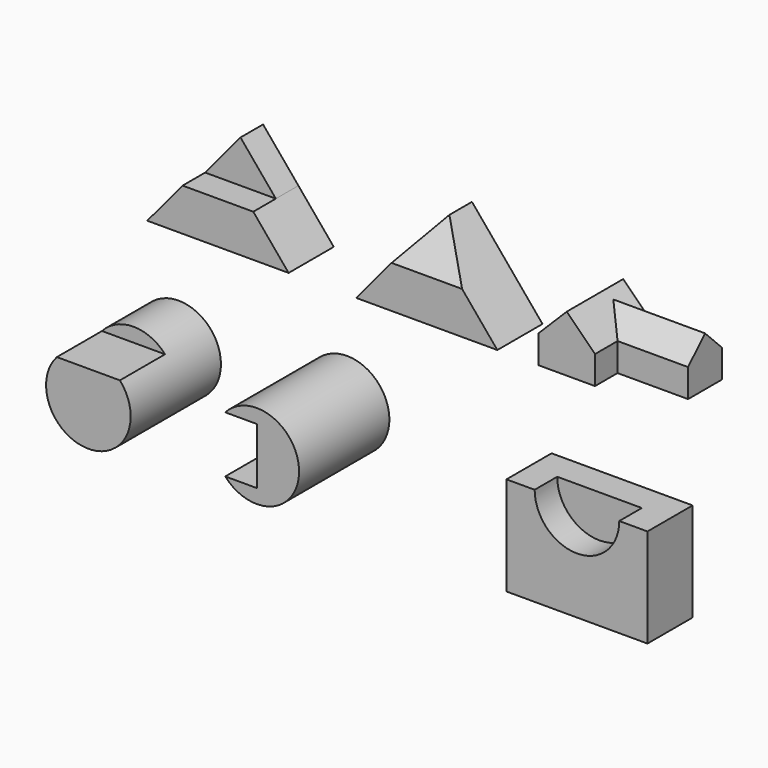
from build123d import *

# Parameters (mm, degrees)
F1_DEPTH  = 101.6
F2_DEPTH  = 50.8
F3_DEPTH  = 101.6
F7_DEPTH  = 63.5
F9_DEPTH  = 127
F12_DEPTH = 165.1
F13_R     = 76.2
F14_DEPTH = 203.2
F16_DEPTH = 101.6
F18_DEPTH = 203.2
F20_DEPTH = 101.6
F21_W     = 254
F21_H     = 177.8
F22_DEPTH = 101.6
F24_DEPTH = 50.8


with BuildPart() as f1:
    # F0 (on Front) → F1 (new body)
    with BuildSketch(Plane.XZ):
        Polygon((275.9973074218, 152.7659382395), (212.3448331553, 76.3829691198), (339.6497816883, 76.3829691198), align=None)
        Polygon((212.3448331553, 76.3829691198), (148.6923588888, 0), (403.3022559547, 0), (339.6497816883, 76.3829691198), align=None)
    extrude(amount=-F1_DEPTH)

    # F0 (on Front) → F2 (cut)
    with BuildSketch(Plane.XZ):
        Polygon((275.9973074218, 152.7659382395), (212.3448331553, 76.3829691198), (339.6497816883, 76.3829691198), align=None)
    extrude(amount=-F2_DEPTH, mode=Mode.SUBTRACT)


with BuildPart() as f3:
    # F0 (on Front) → F3 (new body)
    with BuildSketch(Plane.XZ):
        Polygon((652.2500761549, 152.4), (588.7500761549, 76.2), (715.7500761549, 76.2), align=None)
        Polygon((588.7500761549, 76.2), (525.2500761549, 0), (779.2500761549, 0), (715.7500761549, 76.2), align=None)
    extrude(amount=-F3_DEPTH)

    # F6 (on 3pt) → F7 (cut, symmetric)
    with BuildSketch(Plane.YZ.offset(652.2500761549)):
        Polygon((0, 152.4), (0, 76.2), (50.8, 152.4), align=None)
    extrude(amount=F7_DEPTH, both=True, mode=Mode.SUBTRACT)


with BuildPart() as f9:
    # F8 (on Front) → F9 (new body)
    with BuildSketch(Plane.XZ):
        Polygon((853.4919664163, 50.8), (853.4919664163, 0), (955.0919664163, 0), (955.0919664163, 50.8), (904.2919664163, 101.6), align=None)
    extrude(amount=-F9_DEPTH)

    # F11 (on offset) → F12 (join)
    with BuildSketch(Plane.YZ.offset(1082.0919664163)):
        Polygon((50.8, 0), (127, 0), (127, 50.8), (88.9, 88.9), (50.8, 50.8), align=None)
    extrude(amount=-F12_DEPTH)


with BuildPart() as f14:
    # F13 (on Front) → F14 (new body)
    with BuildSketch(Plane.XZ):
        with Locations((205.21299541, -184.5077127218)):
            Circle(F13_R)
    extrude(amount=F14_DEPTH)

    # F15 (on face) → F16 (cut)
    with BuildSketch(Plane.XZ.offset(203.2)):
        with BuildLine():
            Line((148.4525080283, -133.667894939), (202.7499394524, -133.667894939))
            Line((202.7499394524, -133.667894939), (261.9734827917, -133.667894939))
            ThreePointArc((261.9734827917, -133.667894939), (205.21299541, -108.3077127218), (148.4525080283, -133.667894939))
        make_face()
    extrude(amount=-F16_DEPTH, mode=Mode.SUBTRACT)


with BuildPart() as f18:
    # F17 (on Front) → F18 (new body)
    with BuildSketch(Plane.XZ):
        with BuildLine():
            ThreePointArc((451.7231056446, -224.286083746), (535.7090755138, -244.6700174989), (584.7192322731, -173.486083746))
            ThreePointArc((584.7192322731, -173.486083746), (535.7090755138, -102.302149993), (451.7231056446, -122.686083746))
            Line((451.7231056446, -122.686083746), (508.5192322731, -122.686083746))
            Line((508.5192322731, -122.686083746), (508.5192322731, -224.286083746))
            Line((508.5192322731, -224.286083746), (451.7231056446, -224.286083746))
        make_face()
        with BuildLine():
            Line((508.5192322731, -122.686083746), (451.7231056446, -122.686083746))
            ThreePointArc((451.7231056446, -122.686083746), (432.3192322731, -173.486083746), (451.7231056446, -224.286083746))
            Line((451.7231056446, -224.286083746), (508.5192322731, -224.286083746))
            Line((508.5192322731, -224.286083746), (508.5192322731, -122.686083746))
        make_face()
    extrude(amount=F18_DEPTH)

    # F19 (on face) → F20 (cut)
    with BuildSketch(Plane.XZ.offset(203.2)):
        with BuildLine():
            Line((508.5192322731, -224.286083746), (508.5192322731, -122.686083746))
            Line((508.5192322731, -122.686083746), (451.7231056446, -122.686083746))
            ThreePointArc((451.7231056446, -122.686083746), (432.3192322731, -173.486083746), (451.7231056446, -224.286083746))
            Line((451.7231056446, -224.286083746), (508.5192322731, -224.286083746))
        make_face()
    extrude(amount=-F20_DEPTH, mode=Mode.SUBTRACT)


with BuildPart() as f22:
    # F21 (on Front) → F22 (new body)
    with BuildSketch(Plane.XZ):
        with Locations((1003.8928091526, -220.871200853)):
            Rectangle(F21_W, F21_H)
    extrude(amount=F22_DEPTH)

    # F23 (on face) → F24 (cut)
    with BuildSketch(Plane.XZ.offset(101.6)):
        with BuildLine():
            Line((1080.0928091526, -131.971200853), (927.6928091526, -131.971200853))
            ThreePointArc((927.6928091526, -131.971200853), (1003.8928091526, -208.171200853), (1080.0928091526, -131.971200853))
        make_face()
    extrude(amount=-F24_DEPTH, mode=Mode.SUBTRACT)


solid = Compound([f1.part, f3.part, f9.part, f14.part, f18.part, f22.part])
